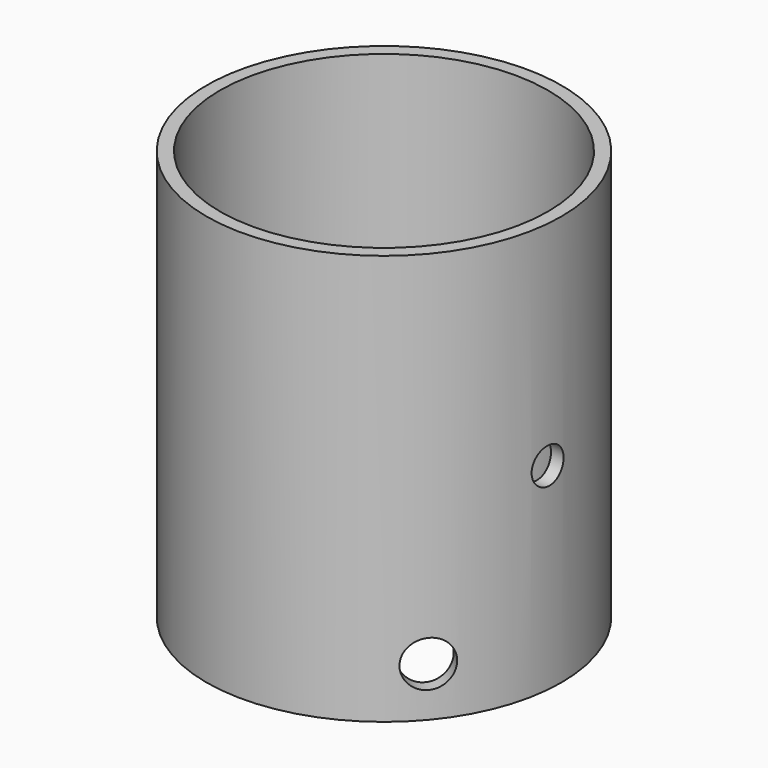
from build123d import *

# Parameters (mm, degrees)
F0_R     = 108.15
F0_R_2   = 99.95
F1_DEPTH = 250
F3_R     = 14
F4_REACH = 191.9641662574
F6_R     = 11
F7_REACH = 148.2780486573


with BuildPart() as f1:
    # F0 (on Top) → F1 (new body)
    with BuildSketch(Plane.XY):
        Circle(F0_R)
        Circle(F0_R_2, mode=Mode.SUBTRACT)
    extrude(amount=F1_DEPTH)

    f4_end = f1.faces().sort_by_distance((-108.15, 0, 125))[0]
    # F3 (on face) → F4 (cut, up to a face of the model that its end follows)
    with BuildSketch(Plane(origin=(0, 0, 0), x_dir=(-0.6427876097, -0.7660444431, 0), z_dir=(-0.7660444431, 0.6427876097, 0))):
        with Locations((0, 30)):
            Circle(F3_R)
    f4_long = extrude(amount=-F4_REACH, mode=Mode.PRIVATE)
    add(split(f4_long, bisect_by=f4_end, keep=Keep.BOTTOM, mode=Mode.PRIVATE), mode=Mode.SUBTRACT)

    f7_end = f1.faces().sort_by_distance((-108.15, 0, 125))[0]
    # F6 (on face) → F7 (cut, up to a face of the model that its end follows)
    with BuildSketch(Plane(origin=(0, 0, 0), x_dir=(-0.0871557427, -0.9961946981, 0), z_dir=(-0.9961946981, 0.0871557427, 0))):
        with Locations((0, 120)):
            Circle(F6_R)
    f7_long = extrude(amount=-F7_REACH, mode=Mode.PRIVATE)
    add(split(f7_long, bisect_by=f7_end, keep=Keep.BOTTOM, mode=Mode.PRIVATE), mode=Mode.SUBTRACT)


solid = f1.part
